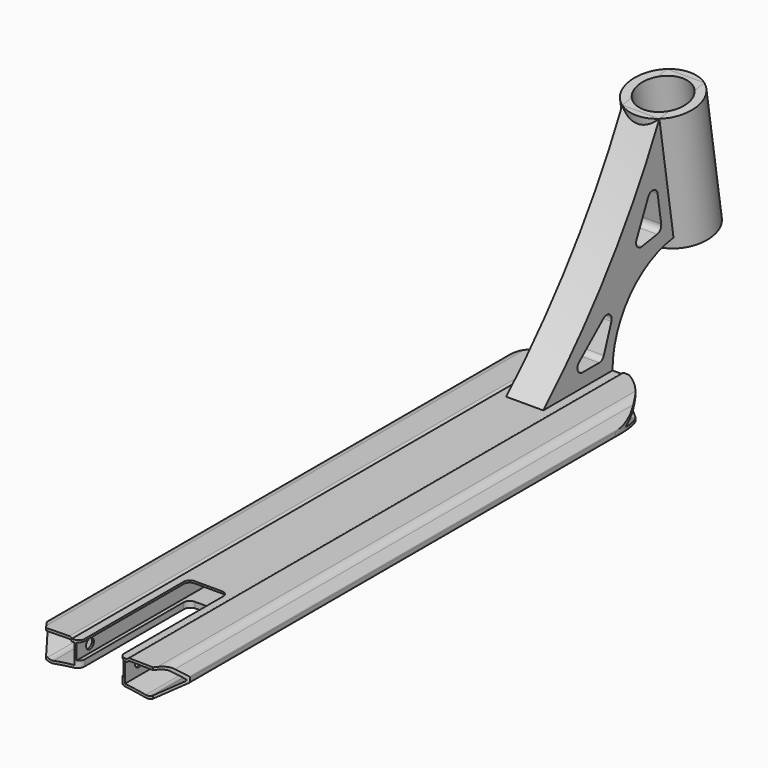
from build123d import *

# Parameters (mm, degrees)
F1_DEPTH       = 250
F2_W           = 38
F2_H           = 13
F3_DEPTH       = 250
F4_T1_DEPTH    = 509.4719116023
F5_R           = 9
F6_R           = 1
F8_DEPTH       = 500.001
F8_DEPTH_BACK  = 764
F10_DEPTH      = 22.6480929268
F10_DEPTH_BACK = 1.2707367785
F12_DEPTH      = 1.2707367785
F12_DEPTH_BACK = 22.6480930395
F13_T1_DEPTH   = 1.6250010516
F13_T6_DEPTH   = 31.6250010516
F13_S7_R       = 200
F13_T8_DEPTH   = 18
F13_T13_DEPTH  = 35.0672691255
F13_S14_R      = 200
F13_T15_DEPTH  = 19
F13_T19_DEPTH  = 65.0672691255
F13_T25_DEPTH  = 31.6250010516
F13_S26_R      = 200
F13_T27_DEPTH  = 18
F13_T32_DEPTH  = 35.0672691255
F13_S33_R      = 200
F13_T34_DEPTH  = 19
F13_T38_DEPTH  = 65.0672691255
F13_T41_DEPTH  = 65.0672691255
F15_DEPTH      = 15
F16_R          = 27.5
F17_DEPTH      = 100
F20_D          = 40
F22_D          = 8
F22_DEPTH      = 77.9752291788
F24_DEPTH      = 72.5010001
F25_R          = 5


# Not quite as in the source:
# - a fillet or chamfer that OpenCascade refuses, or shapes differently, is made with other operations: its cross-section is extruded or revolved along the edge and cut away or added
# - an extrude ends at something that could not be found from the text; its depth is read off the source's solid


with BuildPart() as f1:
    # F0 (on Front) → F1 (new body, symmetric)
    with BuildSketch(Plane.XZ):
        with BuildLine():
            Line((0, 0), (-22.5, 0))
            Line((-22.5, 0), (-22.5, 1.3))
            Line((-22.5, 1.3), (-49.1090036882, 0.8712122544))
            Line((-49.1090036882, 0.8712122544), (-57.5, -9.1287877456))
            Line((-57.5, -9.1287877456), (-57.5, -13.1287877456))
            Line((-57.5, -13.1287877456), (-40.1794919243, -23.1287877456))
            ThreePointArc((-40.1794919243, -23.1287877456), (0, -19.0512428871), (40.1794919243, -23.1287877456))
            Line((40.1794919243, -23.1287877456), (57.5, -13.1287877456))
            Line((57.5, -13.1287877456), (57.5, -9.1287877456))
            Line((57.5, -9.1287877456), (49.1090036882, 0.8712122544))
            Line((49.1090036882, 0.8712122544), (22.5, 1.3))
            Line((22.5, 1.3), (22.5, 0))
            Line((22.5, 0), (0, 0))
        make_face()
    extrude(amount=F1_DEPTH, both=True)

    # F2 (on Front) → F3 (cut, symmetric)
    with BuildSketch(Plane.XZ):
        with Locations((0, -8.1250010516)):
            Rectangle(F2_W, F2_H)
    extrude(amount=F3_DEPTH, both=True, mode=Mode.SUBTRACT)

    # F4: fillet of radius 2 on 2 edges, made by hand

    # F4_s2 → F4_t1 (cut)
    with BuildSketch(Plane.XZ.offset(-254.7359558012)):
        with BuildLine():
            ThreePointArc((-22.5, 0), (-23.2484344275, 0.931112141), (-24.394136408, 1.2694771556))
            Line((-24.394136408, 1.2694771556), (-22.5, 1.3))
            Line((-22.5, 1.3), (-22.5, 0))
        make_face()
        with BuildLine():
            ThreePointArc((24.394136408, 1.2694771556), (23.2484344275, 0.931112141), (22.5, 0))
            Line((22.5, 0), (22.5, 1.3))
            Line((22.5, 1.3), (24.394136408, 1.2694771556))
        make_face()
    extrude(amount=F4_T1_DEPTH, mode=Mode.SUBTRACT)

    # F5
    f5_edges = [f1.edges().sort_by_distance(p)[0] for p in [
        (-49.109004, 0, 0.871212),
        (49.109004, 0, 0.871212),
        (40.179492, 0, -23.128788),
        (-40.179492, 0, -23.128788),
    ]]
    fillet(f5_edges, radius=F5_R)

    # F6
    f6_edges = [f1.edges().sort_by_distance(p)[0] for p in [
        (-57.5, 0, -9.128788),
        (-57.5, 0, -13.128788),
        (57.5, 0, -13.128788),
        (57.5, 0, -9.128788),
    ]]
    fillet(f6_edges, radius=F6_R)

    # F7 (on face) → F8 (cut, two sides)
    with BuildSketch(Plane.XZ.offset(250)) as f8_sk:
        with BuildLine():
            Line((-24.3619118205, -0.7302632216), (-44.9684899588, -1.0623255674))
            ThreePointArc((-44.9684899588, -1.0623255674), (-47.8650468263, -1.7413017644), (-50.2180150044, -3.5619036195))
            Line((-50.2180150044, -3.5619036195), (-55.9308095341, -10.3701470241))
            ThreePointArc((-55.9308095341, -10.3701470241), (-56.149572844, -11.1865828114), (-55.664765091, -11.8789600375))
            Line((-55.664765091, -11.8789600375), (-42.1022690923, -19.7092707533))
            ThreePointArc((-42.1022690923, -19.7092707533), (-39.7790673433, -20.5474658063), (-37.3093701274, -20.526657758))
            ThreePointArc((-37.3093701274, -20.526657758), (-28.9174436166, -19.1318054763), (-20.4742290788, -18.091530647))
            Line((-20.4742290788, -18.091530647), (-20.4742290788, -1.9519160667))
            Line((-20.4742290788, -1.9519160667), (-22.4739694559, -1.9841406542))
            ThreePointArc((-22.4739694559, -1.9841406542), (-23.2231909578, -1.0639705879), (-24.3619118205, -0.7302632216))
        make_face()
        with BuildLine():
            ThreePointArc((24.3619118205, -0.7302632216), (23.2231909578, -1.0639705879), (22.4739694559, -1.9841406542))
            Line((22.4739694559, -1.9841406542), (20.4742290788, -1.9519160667))
            Line((20.4742290788, -1.9519160667), (20.4742290788, -18.091530647))
            ThreePointArc((20.4742290788, -18.091530647), (28.9174436166, -19.1318054763), (37.3093701274, -20.526657758))
            ThreePointArc((37.3093701274, -20.526657758), (39.7790673433, -20.5474658063), (42.1022690923, -19.7092707533))
            Line((42.1022690923, -19.7092707533), (55.664765091, -11.8789600375))
            ThreePointArc((55.664765091, -11.8789600375), (56.149572844, -11.1865828114), (55.9308095341, -10.3701470241))
            Line((55.9308095341, -10.3701470241), (50.2180150044, -3.5619036195))
            ThreePointArc((50.2180150044, -3.5619036195), (47.8650468263, -1.7413017644), (44.9684899588, -1.0623255674))
            Line((44.9684899588, -1.0623255674), (24.3619118205, -0.7302632216))
        make_face()
    extrude(amount=-F8_DEPTH, mode=Mode.SUBTRACT)
    extrude(f8_sk.sketch, amount=F8_DEPTH_BACK, mode=Mode.SUBTRACT)

    # F9 (on Top) → F10 (cut, two sides)
    with BuildSketch(Plane.XY) as f10_sk:
        with BuildLine():
            ThreePointArc((-57.5, 200), (0, 257.5), (57.5, 200))
            Line((57.5, 200), (57.5, 280))
            Line((57.5, 280), (-57.5, 280))
            Line((-57.5, 280), (-57.5, 200))
        make_face()
    extrude(amount=-F10_DEPTH, mode=Mode.SUBTRACT)
    extrude(f10_sk.sketch, amount=F10_DEPTH_BACK, mode=Mode.SUBTRACT)

    # F11 (on Top) → F12 (cut, two sides)
    with BuildSketch(Plane.XY) as f12_sk:
        Polygon((-43.2975540478, -250), (-68, -216), (-68, -346), (68, -346), (68, -216), (43.2975540478, -250), (16, -250), (16, -140), (-16, -140), (-16, -250), align=None)
    extrude(amount=F12_DEPTH, mode=Mode.SUBTRACT)
    extrude(f12_sk.sketch, amount=-F12_DEPTH_BACK, mode=Mode.SUBTRACT)

    # F13: fillet of radius 5 on 6 edges, made by hand

    # F13_s2 → F13_t1 (join)
    with BuildSketch(Plane.XY.offset(-1.6250010516)):
        with BuildLine():
            ThreePointArc((-11, -140), (-14.5355339059, -141.4644660941), (-16, -145))
            Line((-16, -145), (-16.1, -145))
            Line((-16.1, -145), (-16.1, -139.9))
            Line((-16.1, -139.9), (-11, -139.9))
            Line((-11, -139.9), (-11, -140))
        make_face()
        with BuildLine():
            ThreePointArc((16, -145), (14.5355339059, -141.4644660941), (11, -140))
            Line((11, -140), (11, -139.9))
            Line((11, -139.9), (16.1, -139.9))
            Line((16.1, -139.9), (16.1, -145))
            Line((16.1, -145), (16, -145))
        make_face()
    extrude(amount=F13_T1_DEPTH)


with BuildPart() as f13_tool4:
    # F13_s5 → F13_t6 (new body)
    with BuildSketch(Plane.XY.offset(-31.6250010516)):
        with BuildLine():
            ThreePointArc((-11, -140), (-14.5355339059, -141.4644660941), (-16, -145))
            Line((-16, -145), (-16.1, -145))
            Line((-16.1, -145), (-16.1, -139.9))
            Line((-16.1, -139.9), (-11, -139.9))
            Line((-11, -139.9), (-11, -140))
        make_face()
    extrude(amount=F13_T6_DEPTH)

    # F13_s7 → F13_t8 (cut, symmetric)
    with BuildSketch(Plane.XZ.offset(142.4)):
        with Locations((0, -219.0512428871)):
            Circle(F13_S7_R)
    extrude(amount=F13_T8_DEPTH, both=True, mode=Mode.SUBTRACT)

    split(bisect_by=Plane.XY.offset(-14.6250010516), keep=Keep.BOTTOM)


with BuildPart() as f1_1:
    add(f1.part)

    # F13_t3: union F13_tool4
    add(f13_tool4.part)


with BuildPart() as f13_tool11:
    # F13_s12 → F13_t13 (new body)
    with BuildSketch(Plane.XY.offset(-49.6922701771)):
        with BuildLine():
            ThreePointArc((-16, -145), (-14.5355339059, -141.4644660941), (-11, -140))
            Line((-11, -140), (-11, -139.9))
            Line((-11, -139.9), (-16.1, -139.9))
            Line((-16.1, -139.9), (-16.1, -145))
            Line((-16.1, -145), (-16, -145))
        make_face()
    extrude(amount=F13_T13_DEPTH)

    # F13_s14 → F13_t15 (cut, symmetric)
    with BuildSketch(Plane.XZ.offset(142.4)):
        with Locations((0, -219.0512428871)):
            Circle(F13_S14_R)
    extrude(amount=F13_T15_DEPTH, both=True, mode=Mode.SUBTRACT)


with BuildPart() as f1_2:
    add(f1_1.part)

    # F13_t10: union F13_tool11
    add(f13_tool11.part)


with BuildPart() as f13_tool17:
    # F13_s18 → F13_t19 (new body)
    with BuildSketch(Plane.XY.offset(-49.6922701771)):
        with BuildLine():
            ThreePointArc((-16, -145), (-14.5355339059, -141.4644660941), (-11, -140))
            Line((-11, -140), (-11, -139.9))
            Line((-11, -139.9), (-16.1, -139.9))
            Line((-16.1, -139.9), (-16.1, -145))
            Line((-16.1, -145), (-16, -145))
        make_face()
    extrude(amount=F13_T19_DEPTH)

    split(bisect_by=Plane.XY, keep=Keep.BOTTOM)

    split(bisect_by=Plane.XY.offset(-1.6250010516), keep=Keep.TOP)


with BuildPart() as f1_3:
    add(f1_2.part)

    # F13_t16: union F13_tool17
    add(f13_tool17.part)


with BuildPart() as f13_tool23:
    # F13_s24 → F13_t25 (new body)
    with BuildSketch(Plane.XY.offset(-31.6250010516)):
        with BuildLine():
            ThreePointArc((16, -145), (14.5355339059, -141.4644660941), (11, -140))
            Line((11, -140), (11, -139.9))
            Line((11, -139.9), (16.1, -139.9))
            Line((16.1, -139.9), (16.1, -145))
            Line((16.1, -145), (16, -145))
        make_face()
    extrude(amount=F13_T25_DEPTH)

    # F13_s26 → F13_t27 (cut, symmetric)
    with BuildSketch(Plane.XZ.offset(142.4)):
        with Locations((0, -219.0512428871)):
            Circle(F13_S26_R)
    extrude(amount=F13_T27_DEPTH, both=True, mode=Mode.SUBTRACT)

    split(bisect_by=Plane.XY.offset(-14.6250010516), keep=Keep.BOTTOM)


with BuildPart() as f1_4:
    add(f1_3.part)

    # F13_t22: union F13_tool23
    add(f13_tool23.part)


with BuildPart() as f13_tool30:
    # F13_s31 → F13_t32 (new body)
    with BuildSketch(Plane.XY.offset(-49.6922701771)):
        with BuildLine():
            ThreePointArc((11, -140), (14.5355339059, -141.4644660941), (16, -145))
            Line((16, -145), (16.1, -145))
            Line((16.1, -145), (16.1, -139.9))
            Line((16.1, -139.9), (11, -139.9))
            Line((11, -139.9), (11, -140))
        make_face()
    extrude(amount=F13_T32_DEPTH)

    # F13_s33 → F13_t34 (cut, symmetric)
    with BuildSketch(Plane.XZ.offset(142.4)):
        with Locations((0, -219.0512428871)):
            Circle(F13_S33_R)
    extrude(amount=F13_T34_DEPTH, both=True, mode=Mode.SUBTRACT)


with BuildPart() as f1_5:
    add(f1_4.part)

    # F13_t29: union F13_tool30
    add(f13_tool30.part)


with BuildPart() as f13_tool36:
    # F13_s37 → F13_t38 (new body)
    with BuildSketch(Plane.XY.offset(-49.6922701771)):
        with BuildLine():
            ThreePointArc((11, -140), (14.5355339059, -141.4644660941), (16, -145))
            Line((16, -145), (16.1, -145))
            Line((16.1, -145), (16.1, -139.9))
            Line((16.1, -139.9), (11, -139.9))
            Line((11, -139.9), (11, -140))
        make_face()
    extrude(amount=F13_T38_DEPTH)

    split(bisect_by=Plane.XY, keep=Keep.BOTTOM)

    split(bisect_by=Plane.XY.offset(-1.6250010516), keep=Keep.TOP)


with BuildPart() as f1_6:
    add(f1_5.part)

    # F13_t35: union F13_tool36
    add(f13_tool36.part)

    # F13_s42 → F13_t41 (cut)
    with BuildSketch(Plane.XY.offset(-49.6922701771)):
        with BuildLine():
            ThreePointArc((16, -245), (17.4644660941, -248.5355339059), (21, -250))
            Line((21, -250), (21, -250.1))
            Line((21, -250.1), (15.9, -250.1))
            Line((15.9, -250.1), (15.9, -245))
            Line((15.9, -245), (16, -245))
        make_face()
        with BuildLine():
            ThreePointArc((-21, -250), (-17.4644660941, -248.5355339059), (-16, -245))
            Line((-16, -245), (-15.9, -245))
            Line((-15.9, -245), (-15.9, -250.1))
            Line((-15.9, -250.1), (-21, -250.1))
            Line((-21, -250.1), (-21, -250))
        make_face()
    extrude(amount=F13_T41_DEPTH, mode=Mode.SUBTRACT)

    # F14 (on Right) → F15 (join, symmetric)
    with BuildSketch(Plane.YZ):
        with BuildLine():
            ThreePointArc((297.3819995028, 160), (245.9666940414, 74.662277853), (180, 0))
            Line((180, 0), (250, 0))
            ThreePointArc((250, 0), (267.6550746197, 46.4758946867), (311.7145367693, 69.5079211245))
            Line((311.7145367693, 69.5079211245), (312.8715711262, 62.2026937014))
            Line((312.8715711262, 62.2026937014), (313.0254460068, 61.2311659405))
            Line((313.0254460068, 61.2311659405), (358.4591096742, 68.4271513323))
            Line((358.4591096742, 68.4271513323), (342.8156631702, 167.1959853919))
            Line((342.8156631702, 167.1959853919), (297.3819995028, 160))
        make_face()
    extrude(amount=F15_DEPTH, both=True)

    # F16 (on face) → F17 (join, through all)
    with BuildSketch(Plane(origin=(0, -17.4439040266, 110.1364754698), x_dir=(1, 0, 0), z_dir=(0, -0.156434465, 0.9876883406))):
        with Locations((-0.0748134317, 341.7502480182)):
            Circle(F16_R)
    extrude(amount=-F17_DEPTH)

    # F20 (through all)
    with Locations(Plane(origin=(0, -17.4439040266, 110.1364754698), x_dir=(1, 0, 0), z_dir=(0, -0.156434465, 0.9876883406))):
        with Locations((-0.0748134317, 341.7502480182)):
            Hole(F20_D / 2)

    # F22 (through all, one way)
    with BuildSketch(Plane.YZ.offset(20.4742290788)):
        with Locations((-235.9722796521, -8.091530647)):
            Circle(F22_D / 2)
    extrude(amount=-F22_DEPTH, mode=Mode.SUBTRACT)

    # F23 (on face) → F24 (cut, through all)
    with BuildSketch(Plane.YZ.offset(15)):
        Polygon((300.0198733001, 79.4205881019), (292.9803223733, 123.8665634287), (270.3892230822, 74.7275541507), align=None)
        Polygon((240, 10.9374148098), (255.3909064497, 53.2235827452), (206, 10.9374148098), align=None)
    extrude(amount=-F24_DEPTH, mode=Mode.SUBTRACT)

    # F25
    f25_edges = [f1_6.edges().sort_by_distance(p)[0] for p in [
        (0, 240, 10.937415),
        (0, 300.019873, 79.420588),
        (0, 206, 10.937415),
        (0, 270.389223, 74.727554),
        (0, 292.980322, 123.866563),
        (0, 255.390906, 53.223583),
    ]]
    fillet(f25_edges, radius=F25_R)


solid = f1_6.part
